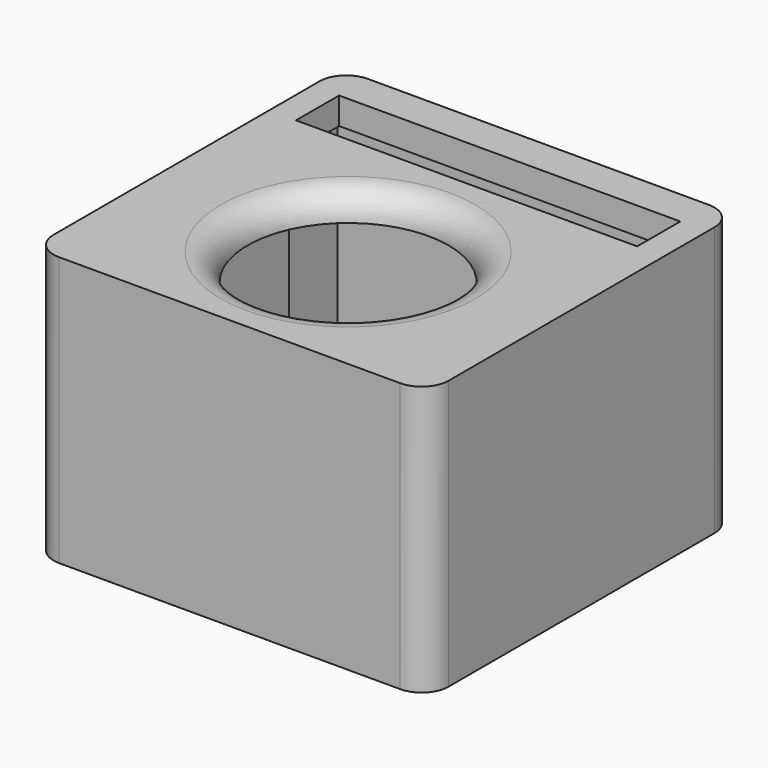
from build123d import *

# Parameters (mm, degrees)
F1_DEPTH = 190.5
F2_W     = 50.8
F2_H     = 19.05
F3_DEPTH = 6.35
F4_W     = 50.8
F4_H     = 19.05
F5_DEPTH = 6.35
F0_W     = 241.3
F0_H     = 184.15
F0_R     = 71
F0_H_2   = 38.1
F6_DEPTH = 19.05
F7_R     = 19.04999


# Not quite as in the source:
# - a fillet or chamfer is up to 0.001 mm smaller than in the source, because OpenCascade refuses the exact size


with BuildPart() as f1:
    # F0 (on Top) → F1 (new body)
    with BuildSketch(Plane.XY):
        with BuildLine():
            Line((-120.65, -136.525), (120.65, -136.525))
            ThreePointArc((120.65, -136.525), (134.1203841816, -130.9453841816), (139.7, -117.475))
            Line((139.7, -117.475), (139.7, 117.475))
            Line((139.7, 117.475), (127, 117.475))
            Line((127, 117.475), (127, 66.675))
            Line((127, 66.675), (120.65, 66.675))
            Line((120.65, 66.675), (120.65, -117.475))
            Line((120.65, -117.475), (-120.65, -117.475))
            Line((-120.65, -117.475), (-120.65, 66.675))
            Line((-120.65, 66.675), (-127, 66.675))
            Line((-127, 66.675), (-127, 117.475))
            Line((-127, 117.475), (-139.7, 117.475))
            Line((-139.7, 117.475), (-139.7, -117.475))
            ThreePointArc((-139.7, -117.475), (-134.1203841816, -130.9453841816), (-120.65, -136.525))
        make_face()
        with BuildLine():
            Line((127, 117.475), (139.7, 117.475))
            ThreePointArc((139.7, 117.475), (134.1203841816, 130.9453841816), (120.65, 136.525))
            Line((120.65, 136.525), (-120.65, 136.525))
            ThreePointArc((-120.65, 136.525), (-134.1203841816, 130.9453841816), (-139.7, 117.475))
            Line((-139.7, 117.475), (-127, 117.475))
            Line((-127, 117.475), (127, 117.475))
        make_face()
    extrude(amount=-F1_DEPTH)

    # F2 (on face) → F3 (join)
    with BuildSketch(Plane(origin=(127, 0, 0), x_dir=(0, -1, 0), z_dir=(-1, 0, 0))):
        with Locations((-92.075, -9.525)):
            Rectangle(F2_W, F2_H)
    extrude(amount=F3_DEPTH)

    # F4 (on face) → F5 (join)
    with BuildSketch(Plane.YZ.offset(-127)):
        with Locations((92.075, -9.525)):
            Rectangle(F4_W, F4_H)
    extrude(amount=F5_DEPTH)

    # F0 (on Top) → F6 (join)
    with BuildSketch(Plane.XY):
        with Locations((0, -25.4)):
            Rectangle(F0_W, F0_H)
        with Locations((0, -31.75)):
            Circle(F0_R, mode=Mode.SUBTRACT)
        Polygon((127, 66.675), (127, 117.475), (-127, 117.475), (-127, 66.675), (-120.65, 66.675), (120.65, 66.675), align=None)
        with Locations((0, 92.075)):
            Rectangle(F0_W, F0_H_2, mode=Mode.SUBTRACT)
    extrude(amount=-F6_DEPTH)

    # F7 (radius 19.05 in the source; OpenCascade refuses exactly that, so slightly less here)
    f7_edges = [f1.edges().sort_by_distance(p)[0] for p in [
        (-71, -31.75, 0),
    ]]
    fillet(f7_edges, radius=F7_R)


solid = f1.part
